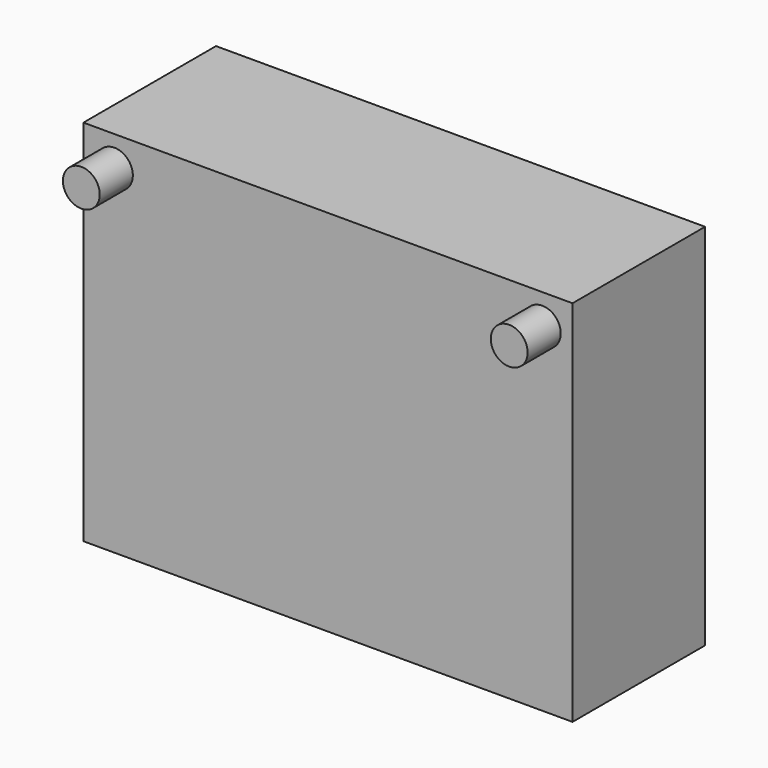
from build123d import *

# Parameters (mm, degrees)
F0_W     = 168.5284674168
F0_H     = 57.090960443
F1_DEPTH = 127
F2_R     = 6.35
F4_DEPTH = 31.75


# Not quite as in the source:
# - the program builds the solid bodies; features that only make, move or delete a surface that nothing else refers to are left out


with BuildPart() as f1:
    # F0 (on Top) → F1 (new body)
    with BuildSketch(Plane.XY):
        with Locations((20.6451192498, 11.0519304872)):
            Rectangle(F0_W, F0_H)
    extrude(amount=F1_DEPTH)

    # F2 (on Front) → F4 (join)
    with BuildSketch(Plane.XZ):
        with Locations((-52.945434434, 116.5131386886)):
            Circle(F2_R)
        with Locations((94.4893505254, 116.5369517954)):
            Circle(F2_R)
    extrude(amount=F4_DEPTH)


solid = f1.part
